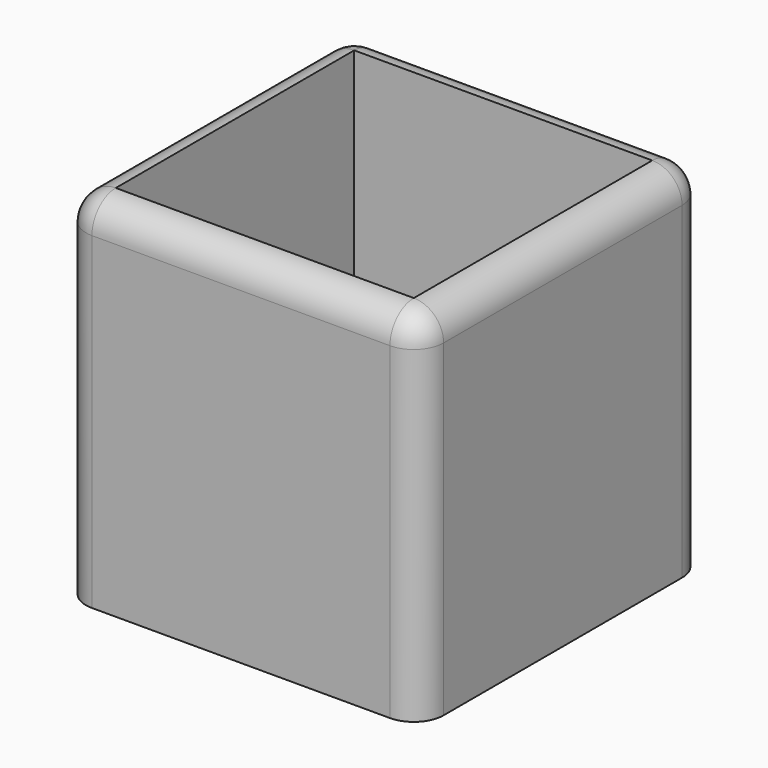
from build123d import *

# Parameters (mm, degrees)
F0_W        = 60
F0_H        = 60
F1_DEPTH    = 60
F2_R        = 5
F3_T1_DEPTH = 67.5
F3_S5_W     = 5
F3_S5_H     = 5
F3_T6_DEPTH = 5
F4_T        = 5
F5_DEPTH    = 12.5


# Not quite as in the source:
# - a fillet or chamfer that OpenCascade refuses, or shapes differently, is made with other operations: its cross-section is extruded or revolved along the edge and cut away or added
# - a shell that OpenCascade refuses in one call is made with other operations: the cavity is built on its own and cut out


with BuildPart() as f1:
    # F0 (on Top) → F1 (new body)
    with BuildSketch(Plane.XY):
        with Locations((17.446616729, -1.6685388982)):
            Rectangle(F0_W, F0_H)
    extrude(amount=F1_DEPTH)

    # F2
    f2_edges = [f1.edges().sort_by_distance(p)[0] for p in [
        (17.446617, -31.668539, 60),
        (47.446617, -1.668539, 60),
        (-12.553383, -1.668539, 60),
        (17.446617, 28.331461, 60),
        (47.446617, 28.331461, 30),
        (47.446617, -31.668539, 30),
        (-12.553383, 28.331461, 30),
    ]]
    fillet(f2_edges, radius=F2_R)

    # F3: fillet of radius 5 on 1 edges, made by hand

    # F3_s2 → F3_t1 (cut)
    with BuildSketch(Plane.XY.offset(-12.5)):
        with BuildLine():
            ThreePointArc((-12.553383271, -26.6685388982), (-11.0889171769, -30.2040728042), (-7.553383271, -31.6685388982))
            Line((-7.553383271, -31.6685388982), (-12.553383271, -31.6685388982))
            Line((-12.553383271, -31.6685388982), (-12.553383271, -26.6685388982))
        make_face()
    extrude(amount=F3_T1_DEPTH, mode=Mode.SUBTRACT)


with BuildPart() as f3_tool4:
    # F3_s5 → F3_t6 (new body)
    with BuildSketch(Plane.YZ.offset(-7.553383271)):
        with Locations((-29.1685388982, 57.5)):
            Rectangle(F3_S5_W, F3_S5_H)
    extrude(amount=-F3_T6_DEPTH)

    # F3_s7 → F3_t8 (revolve, cut)
    with BuildSketch(Plane(origin=(-7.553383271, -26.6685388982, 55), x_dir=(0, 0.7071067812, -0.7071067812), z_dir=(0, 0.7071067812, 0.7071067812))):
        with BuildLine():
            ThreePointArc((0, -5), (5, 0), (0, 5))
            Line((0, 5), (0, -5))
        make_face()
    revolve(axis=Axis((-7.553383271, -26.6685388982, 55), (-1, 0, 0)), mode=Mode.SUBTRACT)


with BuildPart() as f1_1:
    add(f1.part)

    # F3_t3: cut F3_tool4
    add(f3_tool4.part, mode=Mode.SUBTRACT)

    # F4: shell of thickness 5, made by hand


with BuildPart() as f4_core1:
    # F4_t2: copy of F1
    add(f1_1.part)

    # the walls: a layer under each face that stays
    f4_faces = [f4_core1.faces().sort_by_distance(p)[0] for p in [
        (17.446616729, 28.3314611018, 27.5),
        (47.446616729, -1.6685388982, 27.5),
        (17.446616729, -31.6685388982, 27.5),
        (-12.553383271, -1.6685388982, 27.5),
        (17.446616729, -1.6685388982, 60),
    ]]
    thicken(f4_faces, amount=-F4_T, mode=Mode.SUBTRACT)


with BuildPart() as f1_2:
    add(f1_1.part)

    # what is left inside the walls is the cavity
    f4_cavity = [f4_core1.part.solids().sort_by_distance(p)[0] for p in [
        (42.396617, -1.668539, 36.666667),
    ]]
    add(f4_cavity, mode=Mode.SUBTRACT)

    # F5 (cut, symmetric): a face of the model
    f5_faces = [f1_2.faces().sort_by_distance(p)[0] for p in [
        (17.446616729, -1.6685388982, 60),
    ]]
    extrude(f5_faces, amount=F5_DEPTH, both=True, mode=Mode.SUBTRACT)


solid = f1_2.part
